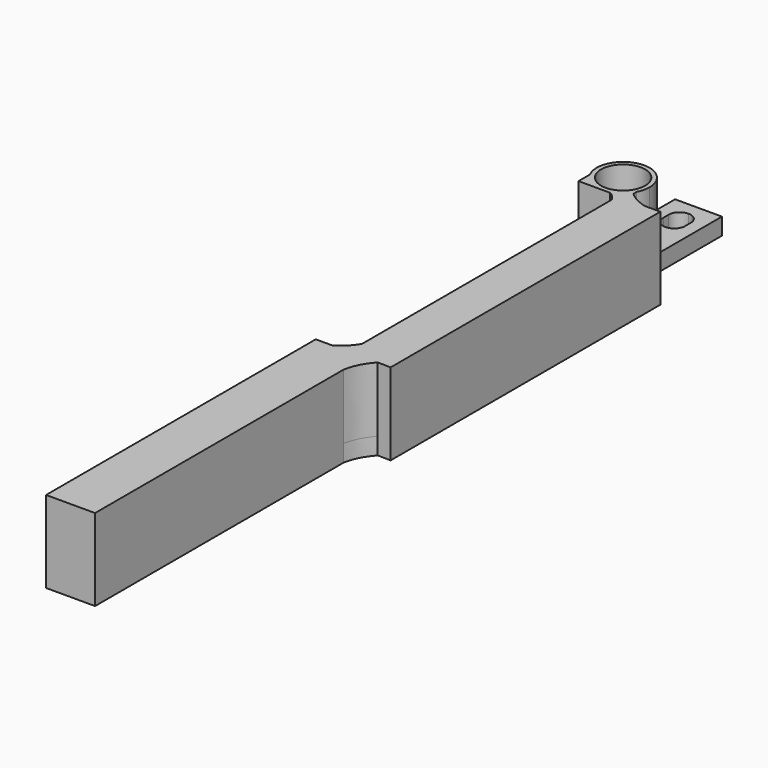
from build123d import *

# Parameters (mm, degrees)
F0_W     = 2.45
F0_H     = 50
F1_DEPTH = 2.5
F2_DEPTH = 9.65
F3_DEPTH = 2.5
F4_DEPTH = 9.65
F5_DEPTH = 9.65
F6_DEPTH = 2.5


with BuildPart() as f1:
    # F0 (on Top) → F1 (new body)
    with BuildSketch(Plane.XY):
        with BuildLine():
            Line((0, 2.1001712409), (0, 0))
            Line((0, 0), (1.025, 0))
            Line((1.025, 0), (1.025, 0.8585484677))
            ThreePointArc((1.025, 0.8585484677), (0.4481513041, 1.426237912), (0, 2.1001712409))
        make_face()
        with BuildLine():
            Line((1.025, 0.8585484677), (1.025, 0))
            Line((1.025, 0), (3.475, 0))
            ThreePointArc((3.475, 0), (2.1769624937, 0.2208504846), (1.025, 0.8585484677))
        make_face()
        with BuildLine():
            ThreePointArc((0, 5.7498287591), (-0.45, 3.925), (0, 2.1001712409))
            Line((0, 2.1001712409), (0, 5.7498287591))
        make_face()
        with BuildLine():
            Line((0, 5.7498287591), (0, 2.1001712409))
            ThreePointArc((0, 2.1001712409), (0.4481513041, 1.426237912), (1.025, 0.8585484677))
            ThreePointArc((1.025, 0.8585484677), (2.1769624937, 0.2208504846), (3.475, 0))
            Line((3.475, 0), (3.475, 0.65))
            ThreePointArc((3.475, 0.65), (0.2, 3.925), (3.475, 7.2))
            Line((3.475, 7.2), (3.475, 7.85))
            ThreePointArc((3.475, 7.85), (1.4448310267, 7.2841723593), (0, 5.7498287591))
        make_face()
        with BuildLine():
            ThreePointArc((5.925, 0.8585484677), (4.7730375063, 0.2208504846), (3.475, 0))
            Line((3.475, 0), (4.7, 0))
            Line((4.7, 0), (5.925, 0))
            Line((5.925, 0), (5.925, 0.8585484677))
        make_face()
        with BuildLine():
            Line((3.475, 0.65), (3.475, 0))
            ThreePointArc((3.475, 0), (4.7730375063, 0.2208504846), (5.925, 0.8585484677))
            ThreePointArc((5.925, 0.8585484677), (6.5018486959, 1.426237912), (6.95, 2.1001712409))
            Line((6.95, 2.1001712409), (6.95, 5.7498287591))
            ThreePointArc((6.95, 5.7498287591), (5.5051689733, 7.2841723593), (3.475, 7.85))
            Line((3.475, 7.85), (3.475, 7.2))
            ThreePointArc((3.475, 7.2), (5.7907747084, 6.2407747084), (6.75, 3.925))
            ThreePointArc((6.75, 3.925), (5.7907747084, 1.6092252916), (3.475, 0.65))
        make_face()
        with BuildLine():
            Line((0, 7.85), (0, 5.7498287591))
            ThreePointArc((0, 5.7498287591), (1.4448310267, 7.2841723593), (3.475, 7.85))
            ThreePointArc((3.475, 7.85), (5.5051689733, 7.2841723593), (6.95, 5.7498287591))
            Line((6.95, 5.7498287591), (6.95, 17.9))
            Line((6.95, 17.9), (3.475, 17.9))
            Line((3.475, 17.9), (0, 17.9))
            Line((0, 17.9), (0, 7.85))
        make_face()
        with BuildLine():
            ThreePointArc((1.8276640256, 14.3833613398), (2.3042302705, 15.55900427), (3.475, 16.0474200003))
            ThreePointArc((3.475, 16.0474200003), (4.5253988967, 15.6691157612), (5.0933824344, 14.7079463483))
            Line((5.0933824344, 14.7079463483), (5.1024433757, 14.1442252627))
            Line((5.1024433757, 14.1442252627), (5.113982201, 13.4263440945))
            ThreePointArc((5.113982201, 13.4263440945), (5.1141409801, 13.4131724726), (5.1141939076, 13.4))
            ThreePointArc((5.1141939076, 13.4), (4.6340851277, 12.2409148723), (3.475, 11.7608060924))
            ThreePointArc((3.475, 11.7608060924), (2.2942628451, 12.2629791393), (1.8369719791, 13.4618131819))
            Line((1.8369719791, 13.4618131819), (1.8276640256, 14.3833613398))
        make_face(mode=Mode.SUBTRACT)
        with BuildLine():
            Line((5.925, 0), (4.7, 0))
            add(Edge.make_bspline(
                [(4.7, 0), (5.2537494339, -0.3164176305), (5.6369397789, -0.7196032093), (5.925, -1.225)],
                knots=[0, 0, 0, 0, 1.7324116139, 1.7324116139, 1.7324116139, 1.7324116139], degree=3))
            Line((5.925, -1.225), (5.925, -0.079424061))
            Line((5.925, -0.079424061), (5.925, 0))
        make_face()
        with BuildLine():
            ThreePointArc((6.95, 2.1001712409), (6.5018486959, 1.426237912), (5.925, 0.8585484677))
            Line((5.925, 0.8585484677), (5.925, 0))
            Line((5.925, 0), (6.95, 0))
            Line((6.95, 0), (6.95, 1.44))
            Line((6.95, 1.44), (6.95, 1.5))
            Line((6.95, 1.5), (6.95, 2.1001712409))
        make_face()
        Polygon((6.95, 0), (5.925, 0), (5.925, -0.079424061), (5.925, -1.225), (5.925, -21.3844068348), (5.925, -22.55), (5.925, -22.9875), (5.925, -25), (9.8284865708, -25), (9.8284865708, -0.079424061), align=None)
        with BuildLine():
            Line((6.95, 5.7498287591), (6.95, 2.1001712409))
            ThreePointArc((6.95, 2.1001712409), (7.2858398025, 2.9852526935), (7.4, 3.925))
            ThreePointArc((7.4, 3.925), (7.2858398025, 4.8647473065), (6.95, 5.7498287591))
        make_face()
        with BuildLine():
            Line((6.95, 1.44), (6.95, 0))
            Line((6.95, 0), (9.8284865708, -0.079424061))
            add(Edge.make_bspline(
                [(6.95, 1.5), (7.7566024847, 0.7003984647), (8.7155010551, 0.2800084476), (9.8284865708, -0.079424061)],
                knots=[0, 0, 0, 0, 3.2833314336, 3.2833314336, 3.2833314336, 3.2833314336], degree=3))
            Line((6.95, 1.5), (6.95, 1.44))
        make_face()
        Polygon((12.1934865708, -0.079424061), (9.8284865708, -0.079424061), (9.8284865708, -25), (9.8284865708, -50.0313035152), (10.2417432854, -50.0397120305), (12.1934865708, -50.079424061), align=None)
        Polygon((9.8284865708, -25), (5.925, -25), (5.925, -26.9515), (5.925, -28.903), (5.925, -47.55), (5.925, -50), (8.29, -50), (9.8284865708, -50.0313035152), align=None)
        with Locations((2.25, -75)):
            Rectangle(F0_W, F0_H)
        with BuildLine():
            Line((10.2417432854, -50.0397120305), (9.8284865708, -50.0313035152))
            Line((9.8284865708, -50.0313035152), (9.8284865708, -50.0397120305))
            Line((9.8284865708, -50.0397120305), (9.8284865708, -50.079424061))
            Line((9.8284865708, -50.079424061), (10.207343012, -50.079424061))
            add(Edge.make_bspline(
                [(10.207343012, -50.079424061), (10.2187605889, -50.0661890592), (10.230227327, -50.0529518896), (10.2417432854, -50.0397120305)],
                knots=[4.2808358806, 4.2808358806, 4.2808358806, 4.2808358806, 4.3292058583, 4.3292058583, 4.3292058583, 4.3292058583], degree=3))
        make_face()
        Polygon((9.8284865708, -50.0397120305), (9.8284865708, -50.0313035152), (8.29, -50), (8.29, -50.0240602729), align=None)
        Polygon((5.925, -50), (3.475, -50), (3.475, -100), (5.925, -100), (5.925, -52.0125), align=None)
        with BuildLine():
            add(Edge.make_bspline(
                [(5.925, -47.55), (5.2342489362, -48.7282052636), (4.4546769932, -49.3181198835), (3.475, -50)],
                knots=[0, 0, 0, 0, 3.4648232278, 3.4648232278, 3.4648232278, 3.4648232278], degree=3))
            Line((3.475, -50), (5.925, -50))
            Line((5.925, -50), (5.925, -47.55))
        make_face()
        with BuildLine():
            Line((9.8284865708, -50.079424061), (9.8284865708, -50.0397120305))
            Line((9.8284865708, -50.0397120305), (8.29, -50.0240602729))
            Line((8.29, -50.0240602729), (8.29, -53.904))
            add(Edge.make_bspline(
                [(8.29, -53.904), (8.5714472143, -52.4050904341), (9.1968655396, -51.250747129), (10.207343012, -50.079424061)],
                knots=[0, 0, 0, 0, 4.2808358806, 4.2808358806, 4.2808358806, 4.2808358806], degree=3))
            Line((10.207343012, -50.079424061), (9.8284865708, -50.079424061))
        make_face()
        Polygon((8.29, -50.0240602729), (8.29, -50), (5.925, -50), align=None)
        Polygon((8.29, -50.0240602729), (5.925, -50), (5.925, -52.0125), (5.925, -100), (8.29, -100), (8.29, -53.904), align=None)
    extrude(amount=-F1_DEPTH)

    # F0 (on Top) → F2 (join)
    with BuildSketch(Plane.XY):
        with BuildLine():
            Line((3.475, 0.65), (3.475, 0))
            ThreePointArc((3.475, 0), (4.7730375063, 0.2208504846), (5.925, 0.8585484677))
            ThreePointArc((5.925, 0.8585484677), (6.5018486959, 1.426237912), (6.95, 2.1001712409))
            Line((6.95, 2.1001712409), (6.95, 5.7498287591))
            ThreePointArc((6.95, 5.7498287591), (5.5051689733, 7.2841723593), (3.475, 7.85))
            Line((3.475, 7.85), (3.475, 7.2))
            ThreePointArc((3.475, 7.2), (5.7907747084, 6.2407747084), (6.75, 3.925))
            ThreePointArc((6.75, 3.925), (5.7907747084, 1.6092252916), (3.475, 0.65))
        make_face()
        with BuildLine():
            Line((0, 5.7498287591), (0, 2.1001712409))
            ThreePointArc((0, 2.1001712409), (0.4481513041, 1.426237912), (1.025, 0.8585484677))
            ThreePointArc((1.025, 0.8585484677), (2.1769624937, 0.2208504846), (3.475, 0))
            Line((3.475, 0), (3.475, 0.65))
            ThreePointArc((3.475, 0.65), (0.2, 3.925), (3.475, 7.2))
            Line((3.475, 7.2), (3.475, 7.85))
            ThreePointArc((3.475, 7.85), (1.4448310267, 7.2841723593), (0, 5.7498287591))
        make_face()
        with BuildLine():
            Line((6.95, 5.7498287591), (6.95, 2.1001712409))
            ThreePointArc((6.95, 2.1001712409), (7.2858398025, 2.9852526935), (7.4, 3.925))
            ThreePointArc((7.4, 3.925), (7.2858398025, 4.8647473065), (6.95, 5.7498287591))
        make_face()
        with BuildLine():
            ThreePointArc((0, 5.7498287591), (-0.45, 3.925), (0, 2.1001712409))
            Line((0, 2.1001712409), (0, 5.7498287591))
        make_face()
        with BuildLine():
            Line((6.95, 1.44), (6.95, 0))
            Line((6.95, 0), (9.8284865708, -0.079424061))
            add(Edge.make_bspline(
                [(6.95, 1.5), (7.7566024847, 0.7003984647), (8.7155010551, 0.2800084476), (9.8284865708, -0.079424061)],
                knots=[0, 0, 0, 0, 3.2833314336, 3.2833314336, 3.2833314336, 3.2833314336], degree=3))
            Line((6.95, 1.5), (6.95, 1.44))
        make_face()
        with BuildLine():
            ThreePointArc((6.95, 2.1001712409), (6.5018486959, 1.426237912), (5.925, 0.8585484677))
            Line((5.925, 0.8585484677), (5.925, 0))
            Line((5.925, 0), (6.95, 0))
            Line((6.95, 0), (6.95, 1.44))
            Line((6.95, 1.44), (6.95, 1.5))
            Line((6.95, 1.5), (6.95, 2.1001712409))
        make_face()
        with BuildLine():
            ThreePointArc((5.925, 0.8585484677), (4.7730375063, 0.2208504846), (3.475, 0))
            Line((3.475, 0), (4.7, 0))
            Line((4.7, 0), (5.925, 0))
            Line((5.925, 0), (5.925, 0.8585484677))
        make_face()
        with BuildLine():
            Line((1.025, 0.8585484677), (1.025, 0))
            Line((1.025, 0), (3.475, 0))
            ThreePointArc((3.475, 0), (2.1769624937, 0.2208504846), (1.025, 0.8585484677))
        make_face()
        with BuildLine():
            Line((0, 2.1001712409), (0, 0))
            Line((0, 0), (1.025, 0))
            Line((1.025, 0), (1.025, 0.8585484677))
            ThreePointArc((1.025, 0.8585484677), (0.4481513041, 1.426237912), (0, 2.1001712409))
        make_face()
        Polygon((6.95, 0), (5.925, 0), (5.925, -0.079424061), (5.925, -1.225), (5.925, -21.3844068348), (5.925, -22.55), (5.925, -22.9875), (5.925, -25), (9.8284865708, -25), (9.8284865708, -0.079424061), align=None)
        with BuildLine():
            Line((5.925, 0), (4.7, 0))
            add(Edge.make_bspline(
                [(4.7, 0), (5.2537494339, -0.3164176305), (5.6369397789, -0.7196032093), (5.925, -1.225)],
                knots=[0, 0, 0, 0, 1.7324116139, 1.7324116139, 1.7324116139, 1.7324116139], degree=3))
            Line((5.925, -1.225), (5.925, -0.079424061))
            Line((5.925, -0.079424061), (5.925, 0))
        make_face()
        Polygon((9.8284865708, -25), (5.925, -25), (5.925, -26.9515), (5.925, -28.903), (5.925, -47.55), (5.925, -50), (8.29, -50), (9.8284865708, -50.0313035152), align=None)
        with BuildLine():
            add(Edge.make_bspline(
                [(5.925, -47.55), (5.2342489362, -48.7282052636), (4.4546769932, -49.3181198835), (3.475, -50)],
                knots=[0, 0, 0, 0, 3.4648232278, 3.4648232278, 3.4648232278, 3.4648232278], degree=3))
            Line((3.475, -50), (5.925, -50))
            Line((5.925, -50), (5.925, -47.55))
        make_face()
        Polygon((8.29, -50.0240602729), (5.925, -50), (5.925, -52.0125), (5.925, -100), (8.29, -100), (8.29, -53.904), align=None)
        Polygon((5.925, -50), (3.475, -50), (3.475, -100), (5.925, -100), (5.925, -52.0125), align=None)
        with Locations((2.25, -75)):
            Rectangle(F0_W, F0_H)
    extrude(amount=F2_DEPTH)

    # F0 (on Top) → F3 (join)
    with BuildSketch(Plane.XY):
        Polygon((12.1934865708, -0.079424061), (9.8284865708, -0.079424061), (9.8284865708, -25), (9.8284865708, -50.0313035152), (10.2417432854, -50.0397120305), (12.1934865708, -50.079424061), align=None)
        Polygon((8.29, -50.0240602729), (5.925, -50), (5.925, -52.0125), (5.925, -100), (8.29, -100), (8.29, -53.904), align=None)
        with BuildLine():
            Line((9.8284865708, -50.079424061), (9.8284865708, -50.0397120305))
            Line((9.8284865708, -50.0397120305), (8.29, -50.0240602729))
            Line((8.29, -50.0240602729), (8.29, -53.904))
            add(Edge.make_bspline(
                [(8.29, -53.904), (8.5714472143, -52.4050904341), (9.1968655396, -51.250747129), (10.207343012, -50.079424061)],
                knots=[0, 0, 0, 0, 4.2808358806, 4.2808358806, 4.2808358806, 4.2808358806], degree=3))
            Line((10.207343012, -50.079424061), (9.8284865708, -50.079424061))
        make_face()
    extrude(amount=-F3_DEPTH)

    # F0 (on Top) → F4 (join)
    with BuildSketch(Plane.XY):
        with BuildLine():
            Line((0, 2.1001712409), (0, 0))
            Line((0, 0), (1.025, 0))
            Line((1.025, 0), (1.025, 0.8585484677))
            ThreePointArc((1.025, 0.8585484677), (0.4481513041, 1.426237912), (0, 2.1001712409))
        make_face()
        with BuildLine():
            Line((1.025, 0.8585484677), (1.025, 0))
            Line((1.025, 0), (3.475, 0))
            ThreePointArc((3.475, 0), (2.1769624937, 0.2208504846), (1.025, 0.8585484677))
        make_face()
        with BuildLine():
            ThreePointArc((0, 5.7498287591), (-0.45, 3.925), (0, 2.1001712409))
            Line((0, 2.1001712409), (0, 5.7498287591))
        make_face()
        with BuildLine():
            Line((0, 5.7498287591), (0, 2.1001712409))
            ThreePointArc((0, 2.1001712409), (0.4481513041, 1.426237912), (1.025, 0.8585484677))
            ThreePointArc((1.025, 0.8585484677), (2.1769624937, 0.2208504846), (3.475, 0))
            Line((3.475, 0), (3.475, 0.65))
            ThreePointArc((3.475, 0.65), (0.2, 3.925), (3.475, 7.2))
            Line((3.475, 7.2), (3.475, 7.85))
            ThreePointArc((3.475, 7.85), (1.4448310267, 7.2841723593), (0, 5.7498287591))
        make_face()
        with BuildLine():
            ThreePointArc((5.925, 0.8585484677), (4.7730375063, 0.2208504846), (3.475, 0))
            Line((3.475, 0), (4.7, 0))
            Line((4.7, 0), (5.925, 0))
            Line((5.925, 0), (5.925, 0.8585484677))
        make_face()
        with BuildLine():
            Line((3.475, 0.65), (3.475, 0))
            ThreePointArc((3.475, 0), (4.7730375063, 0.2208504846), (5.925, 0.8585484677))
            ThreePointArc((5.925, 0.8585484677), (6.5018486959, 1.426237912), (6.95, 2.1001712409))
            Line((6.95, 2.1001712409), (6.95, 5.7498287591))
            ThreePointArc((6.95, 5.7498287591), (5.5051689733, 7.2841723593), (3.475, 7.85))
            Line((3.475, 7.85), (3.475, 7.2))
            ThreePointArc((3.475, 7.2), (5.7907747084, 6.2407747084), (6.75, 3.925))
            ThreePointArc((6.75, 3.925), (5.7907747084, 1.6092252916), (3.475, 0.65))
        make_face()
        with BuildLine():
            Line((5.925, 0), (4.7, 0))
            add(Edge.make_bspline(
                [(4.7, 0), (5.2537494339, -0.3164176305), (5.6369397789, -0.7196032093), (5.925, -1.225)],
                knots=[0, 0, 0, 0, 1.7324116139, 1.7324116139, 1.7324116139, 1.7324116139], degree=3))
            Line((5.925, -1.225), (5.925, -0.079424061))
            Line((5.925, -0.079424061), (5.925, 0))
        make_face()
        with BuildLine():
            ThreePointArc((6.95, 2.1001712409), (6.5018486959, 1.426237912), (5.925, 0.8585484677))
            Line((5.925, 0.8585484677), (5.925, 0))
            Line((5.925, 0), (6.95, 0))
            Line((6.95, 0), (6.95, 1.44))
            Line((6.95, 1.44), (6.95, 1.5))
            Line((6.95, 1.5), (6.95, 2.1001712409))
        make_face()
        Polygon((6.95, 0), (5.925, 0), (5.925, -0.079424061), (5.925, -1.225), (5.925, -21.3844068348), (5.925, -22.55), (5.925, -22.9875), (5.925, -25), (9.8284865708, -25), (9.8284865708, -0.079424061), align=None)
        with BuildLine():
            Line((6.95, 5.7498287591), (6.95, 2.1001712409))
            ThreePointArc((6.95, 2.1001712409), (7.2858398025, 2.9852526935), (7.4, 3.925))
            ThreePointArc((7.4, 3.925), (7.2858398025, 4.8647473065), (6.95, 5.7498287591))
        make_face()
        with BuildLine():
            Line((6.95, 1.44), (6.95, 0))
            Line((6.95, 0), (9.8284865708, -0.079424061))
            add(Edge.make_bspline(
                [(6.95, 1.5), (7.7566024847, 0.7003984647), (8.7155010551, 0.2800084476), (9.8284865708, -0.079424061)],
                knots=[0, 0, 0, 0, 3.2833314336, 3.2833314336, 3.2833314336, 3.2833314336], degree=3))
            Line((6.95, 1.5), (6.95, 1.44))
        make_face()
        Polygon((12.1934865708, -0.079424061), (9.8284865708, -0.079424061), (9.8284865708, -25), (9.8284865708, -50.0313035152), (10.2417432854, -50.0397120305), (12.1934865708, -50.079424061), align=None)
        with BuildLine():
            Line((9.8284865708, -50.079424061), (9.8284865708, -50.0397120305))
            Line((9.8284865708, -50.0397120305), (8.29, -50.0240602729))
            Line((8.29, -50.0240602729), (8.29, -53.904))
            add(Edge.make_bspline(
                [(8.29, -53.904), (8.5714472143, -52.4050904341), (9.1968655396, -51.250747129), (10.207343012, -50.079424061)],
                knots=[0, 0, 0, 0, 4.2808358806, 4.2808358806, 4.2808358806, 4.2808358806], degree=3))
            Line((10.207343012, -50.079424061), (9.8284865708, -50.079424061))
        make_face()
        Polygon((8.29, -50.0240602729), (5.925, -50), (5.925, -52.0125), (5.925, -100), (8.29, -100), (8.29, -53.904), align=None)
    extrude(amount=F4_DEPTH)

    # F0 (on Top) → F5 (join)
    with BuildSketch(Plane.XY):
        with BuildLine():
            Line((0, 2.1001712409), (0, 0))
            Line((0, 0), (1.025, 0))
            Line((1.025, 0), (1.025, 0.8585484677))
            ThreePointArc((1.025, 0.8585484677), (0.4481513041, 1.426237912), (0, 2.1001712409))
        make_face()
        with BuildLine():
            Line((1.025, 0.8585484677), (1.025, 0))
            Line((1.025, 0), (3.475, 0))
            ThreePointArc((3.475, 0), (2.1769624937, 0.2208504846), (1.025, 0.8585484677))
        make_face()
        with BuildLine():
            ThreePointArc((0, 5.7498287591), (-0.45, 3.925), (0, 2.1001712409))
            Line((0, 2.1001712409), (0, 5.7498287591))
        make_face()
        with BuildLine():
            Line((0, 5.7498287591), (0, 2.1001712409))
            ThreePointArc((0, 2.1001712409), (0.4481513041, 1.426237912), (1.025, 0.8585484677))
            ThreePointArc((1.025, 0.8585484677), (2.1769624937, 0.2208504846), (3.475, 0))
            Line((3.475, 0), (3.475, 0.65))
            ThreePointArc((3.475, 0.65), (0.2, 3.925), (3.475, 7.2))
            Line((3.475, 7.2), (3.475, 7.85))
            ThreePointArc((3.475, 7.85), (1.4448310267, 7.2841723593), (0, 5.7498287591))
        make_face()
        with BuildLine():
            ThreePointArc((5.925, 0.8585484677), (4.7730375063, 0.2208504846), (3.475, 0))
            Line((3.475, 0), (4.7, 0))
            Line((4.7, 0), (5.925, 0))
            Line((5.925, 0), (5.925, 0.8585484677))
        make_face()
        with BuildLine():
            Line((3.475, 0.65), (3.475, 0))
            ThreePointArc((3.475, 0), (4.7730375063, 0.2208504846), (5.925, 0.8585484677))
            ThreePointArc((5.925, 0.8585484677), (6.5018486959, 1.426237912), (6.95, 2.1001712409))
            Line((6.95, 2.1001712409), (6.95, 5.7498287591))
            ThreePointArc((6.95, 5.7498287591), (5.5051689733, 7.2841723593), (3.475, 7.85))
            Line((3.475, 7.85), (3.475, 7.2))
            ThreePointArc((3.475, 7.2), (5.7907747084, 6.2407747084), (6.75, 3.925))
            ThreePointArc((6.75, 3.925), (5.7907747084, 1.6092252916), (3.475, 0.65))
        make_face()
        with BuildLine():
            Line((5.925, 0), (4.7, 0))
            add(Edge.make_bspline(
                [(4.7, 0), (5.2537494339, -0.3164176305), (5.6369397789, -0.7196032093), (5.925, -1.225)],
                knots=[0, 0, 0, 0, 1.7324116139, 1.7324116139, 1.7324116139, 1.7324116139], degree=3))
            Line((5.925, -1.225), (5.925, -0.079424061))
            Line((5.925, -0.079424061), (5.925, 0))
        make_face()
        with BuildLine():
            ThreePointArc((6.95, 2.1001712409), (6.5018486959, 1.426237912), (5.925, 0.8585484677))
            Line((5.925, 0.8585484677), (5.925, 0))
            Line((5.925, 0), (6.95, 0))
            Line((6.95, 0), (6.95, 1.44))
            Line((6.95, 1.44), (6.95, 1.5))
            Line((6.95, 1.5), (6.95, 2.1001712409))
        make_face()
        Polygon((6.95, 0), (5.925, 0), (5.925, -0.079424061), (5.925, -1.225), (5.925, -21.3844068348), (5.925, -22.55), (5.925, -22.9875), (5.925, -25), (9.8284865708, -25), (9.8284865708, -0.079424061), align=None)
        with BuildLine():
            Line((6.95, 5.7498287591), (6.95, 2.1001712409))
            ThreePointArc((6.95, 2.1001712409), (7.2858398025, 2.9852526935), (7.4, 3.925))
            ThreePointArc((7.4, 3.925), (7.2858398025, 4.8647473065), (6.95, 5.7498287591))
        make_face()
        with BuildLine():
            Line((6.95, 1.44), (6.95, 0))
            Line((6.95, 0), (9.8284865708, -0.079424061))
            add(Edge.make_bspline(
                [(6.95, 1.5), (7.7566024847, 0.7003984647), (8.7155010551, 0.2800084476), (9.8284865708, -0.079424061)],
                knots=[0, 0, 0, 0, 3.2833314336, 3.2833314336, 3.2833314336, 3.2833314336], degree=3))
            Line((6.95, 1.5), (6.95, 1.44))
        make_face()
        Polygon((12.1934865708, -0.079424061), (9.8284865708, -0.079424061), (9.8284865708, -25), (9.8284865708, -50.0313035152), (10.2417432854, -50.0397120305), (12.1934865708, -50.079424061), align=None)
        Polygon((9.8284865708, -25), (5.925, -25), (5.925, -26.9515), (5.925, -28.903), (5.925, -47.55), (5.925, -50), (8.29, -50), (9.8284865708, -50.0313035152), align=None)
        with Locations((2.25, -75)):
            Rectangle(F0_W, F0_H)
        with BuildLine():
            Line((10.2417432854, -50.0397120305), (9.8284865708, -50.0313035152))
            Line((9.8284865708, -50.0313035152), (9.8284865708, -50.0397120305))
            Line((9.8284865708, -50.0397120305), (9.8284865708, -50.079424061))
            Line((9.8284865708, -50.079424061), (10.207343012, -50.079424061))
            add(Edge.make_bspline(
                [(10.207343012, -50.079424061), (10.2187605889, -50.0661890592), (10.230227327, -50.0529518896), (10.2417432854, -50.0397120305)],
                knots=[4.2808358806, 4.2808358806, 4.2808358806, 4.2808358806, 4.3292058583, 4.3292058583, 4.3292058583, 4.3292058583], degree=3))
        make_face()
        Polygon((9.8284865708, -50.0397120305), (9.8284865708, -50.0313035152), (8.29, -50), (8.29, -50.0240602729), align=None)
        Polygon((5.925, -50), (3.475, -50), (3.475, -100), (5.925, -100), (5.925, -52.0125), align=None)
        with BuildLine():
            add(Edge.make_bspline(
                [(5.925, -47.55), (5.2342489362, -48.7282052636), (4.4546769932, -49.3181198835), (3.475, -50)],
                knots=[0, 0, 0, 0, 3.4648232278, 3.4648232278, 3.4648232278, 3.4648232278], degree=3))
            Line((3.475, -50), (5.925, -50))
            Line((5.925, -50), (5.925, -47.55))
        make_face()
        Polygon((8.29, -50.0240602729), (8.29, -50), (5.925, -50), align=None)
    extrude(amount=F5_DEPTH)

    # F0 (on Top) → F6 (join)
    with BuildSketch(Plane.XY):
        with BuildLine():
            Line((0, 2.1001712409), (0, 0))
            Line((0, 0), (1.025, 0))
            Line((1.025, 0), (1.025, 0.8585484677))
            ThreePointArc((1.025, 0.8585484677), (0.4481513041, 1.426237912), (0, 2.1001712409))
        make_face()
        with BuildLine():
            Line((1.025, 0.8585484677), (1.025, 0))
            Line((1.025, 0), (3.475, 0))
            ThreePointArc((3.475, 0), (2.1769624937, 0.2208504846), (1.025, 0.8585484677))
        make_face()
        with BuildLine():
            ThreePointArc((0, 5.7498287591), (-0.45, 3.925), (0, 2.1001712409))
            Line((0, 2.1001712409), (0, 5.7498287591))
        make_face()
        with BuildLine():
            Line((0, 5.7498287591), (0, 2.1001712409))
            ThreePointArc((0, 2.1001712409), (0.4481513041, 1.426237912), (1.025, 0.8585484677))
            ThreePointArc((1.025, 0.8585484677), (2.1769624937, 0.2208504846), (3.475, 0))
            Line((3.475, 0), (3.475, 0.65))
            ThreePointArc((3.475, 0.65), (0.2, 3.925), (3.475, 7.2))
            Line((3.475, 7.2), (3.475, 7.85))
            ThreePointArc((3.475, 7.85), (1.4448310267, 7.2841723593), (0, 5.7498287591))
        make_face()
        with BuildLine():
            ThreePointArc((5.925, 0.8585484677), (4.7730375063, 0.2208504846), (3.475, 0))
            Line((3.475, 0), (4.7, 0))
            Line((4.7, 0), (5.925, 0))
            Line((5.925, 0), (5.925, 0.8585484677))
        make_face()
        with BuildLine():
            Line((3.475, 0.65), (3.475, 0))
            ThreePointArc((3.475, 0), (4.7730375063, 0.2208504846), (5.925, 0.8585484677))
            ThreePointArc((5.925, 0.8585484677), (6.5018486959, 1.426237912), (6.95, 2.1001712409))
            Line((6.95, 2.1001712409), (6.95, 5.7498287591))
            ThreePointArc((6.95, 5.7498287591), (5.5051689733, 7.2841723593), (3.475, 7.85))
            Line((3.475, 7.85), (3.475, 7.2))
            ThreePointArc((3.475, 7.2), (5.7907747084, 6.2407747084), (6.75, 3.925))
            ThreePointArc((6.75, 3.925), (5.7907747084, 1.6092252916), (3.475, 0.65))
        make_face()
        with BuildLine():
            Line((0, 7.85), (0, 5.7498287591))
            ThreePointArc((0, 5.7498287591), (1.4448310267, 7.2841723593), (3.475, 7.85))
            ThreePointArc((3.475, 7.85), (5.5051689733, 7.2841723593), (6.95, 5.7498287591))
            Line((6.95, 5.7498287591), (6.95, 17.9))
            Line((6.95, 17.9), (3.475, 17.9))
            Line((3.475, 17.9), (0, 17.9))
            Line((0, 17.9), (0, 7.85))
        make_face()
        with BuildLine():
            ThreePointArc((1.8276640256, 14.3833613398), (2.3042302705, 15.55900427), (3.475, 16.0474200003))
            ThreePointArc((3.475, 16.0474200003), (4.5253988967, 15.6691157612), (5.0933824344, 14.7079463483))
            Line((5.0933824344, 14.7079463483), (5.1024433757, 14.1442252627))
            Line((5.1024433757, 14.1442252627), (5.113982201, 13.4263440945))
            ThreePointArc((5.113982201, 13.4263440945), (5.1141409801, 13.4131724726), (5.1141939076, 13.4))
            ThreePointArc((5.1141939076, 13.4), (4.6340851277, 12.2409148723), (3.475, 11.7608060924))
            ThreePointArc((3.475, 11.7608060924), (2.2942628451, 12.2629791393), (1.8369719791, 13.4618131819))
            Line((1.8369719791, 13.4618131819), (1.8276640256, 14.3833613398))
        make_face(mode=Mode.SUBTRACT)
        with BuildLine():
            Line((5.925, 0), (4.7, 0))
            add(Edge.make_bspline(
                [(4.7, 0), (5.2537494339, -0.3164176305), (5.6369397789, -0.7196032093), (5.925, -1.225)],
                knots=[0, 0, 0, 0, 1.7324116139, 1.7324116139, 1.7324116139, 1.7324116139], degree=3))
            Line((5.925, -1.225), (5.925, -0.079424061))
            Line((5.925, -0.079424061), (5.925, 0))
        make_face()
        with BuildLine():
            ThreePointArc((6.95, 2.1001712409), (6.5018486959, 1.426237912), (5.925, 0.8585484677))
            Line((5.925, 0.8585484677), (5.925, 0))
            Line((5.925, 0), (6.95, 0))
            Line((6.95, 0), (6.95, 1.44))
            Line((6.95, 1.44), (6.95, 1.5))
            Line((6.95, 1.5), (6.95, 2.1001712409))
        make_face()
        Polygon((6.95, 0), (5.925, 0), (5.925, -0.079424061), (5.925, -1.225), (5.925, -21.3844068348), (5.925, -22.55), (5.925, -22.9875), (5.925, -25), (9.8284865708, -25), (9.8284865708, -0.079424061), align=None)
        with BuildLine():
            Line((6.95, 5.7498287591), (6.95, 2.1001712409))
            ThreePointArc((6.95, 2.1001712409), (7.2858398025, 2.9852526935), (7.4, 3.925))
            ThreePointArc((7.4, 3.925), (7.2858398025, 4.8647473065), (6.95, 5.7498287591))
        make_face()
        with BuildLine():
            Line((6.95, 1.44), (6.95, 0))
            Line((6.95, 0), (9.8284865708, -0.079424061))
            add(Edge.make_bspline(
                [(6.95, 1.5), (7.7566024847, 0.7003984647), (8.7155010551, 0.2800084476), (9.8284865708, -0.079424061)],
                knots=[0, 0, 0, 0, 3.2833314336, 3.2833314336, 3.2833314336, 3.2833314336], degree=3))
            Line((6.95, 1.5), (6.95, 1.44))
        make_face()
        Polygon((12.1934865708, -0.079424061), (9.8284865708, -0.079424061), (9.8284865708, -25), (9.8284865708, -50.0313035152), (10.2417432854, -50.0397120305), (12.1934865708, -50.079424061), align=None)
        Polygon((9.8284865708, -25), (5.925, -25), (5.925, -26.9515), (5.925, -28.903), (5.925, -47.55), (5.925, -50), (8.29, -50), (9.8284865708, -50.0313035152), align=None)
        with Locations((2.25, -75)):
            Rectangle(F0_W, F0_H)
        with BuildLine():
            Line((10.2417432854, -50.0397120305), (9.8284865708, -50.0313035152))
            Line((9.8284865708, -50.0313035152), (9.8284865708, -50.0397120305))
            Line((9.8284865708, -50.0397120305), (9.8284865708, -50.079424061))
            Line((9.8284865708, -50.079424061), (10.207343012, -50.079424061))
            add(Edge.make_bspline(
                [(10.207343012, -50.079424061), (10.2187605889, -50.0661890592), (10.230227327, -50.0529518896), (10.2417432854, -50.0397120305)],
                knots=[4.2808358806, 4.2808358806, 4.2808358806, 4.2808358806, 4.3292058583, 4.3292058583, 4.3292058583, 4.3292058583], degree=3))
        make_face()
        Polygon((9.8284865708, -50.0397120305), (9.8284865708, -50.0313035152), (8.29, -50), (8.29, -50.0240602729), align=None)
        Polygon((5.925, -50), (3.475, -50), (3.475, -100), (5.925, -100), (5.925, -52.0125), align=None)
        with BuildLine():
            add(Edge.make_bspline(
                [(5.925, -47.55), (5.2342489362, -48.7282052636), (4.4546769932, -49.3181198835), (3.475, -50)],
                knots=[0, 0, 0, 0, 3.4648232278, 3.4648232278, 3.4648232278, 3.4648232278], degree=3))
            Line((3.475, -50), (5.925, -50))
            Line((5.925, -50), (5.925, -47.55))
        make_face()
        with BuildLine():
            Line((9.8284865708, -50.079424061), (9.8284865708, -50.0397120305))
            Line((9.8284865708, -50.0397120305), (8.29, -50.0240602729))
            Line((8.29, -50.0240602729), (8.29, -53.904))
            add(Edge.make_bspline(
                [(8.29, -53.904), (8.5714472143, -52.4050904341), (9.1968655396, -51.250747129), (10.207343012, -50.079424061)],
                knots=[0, 0, 0, 0, 4.2808358806, 4.2808358806, 4.2808358806, 4.2808358806], degree=3))
            Line((10.207343012, -50.079424061), (9.8284865708, -50.079424061))
        make_face()
        Polygon((8.29, -50.0240602729), (8.29, -50), (5.925, -50), align=None)
        Polygon((8.29, -50.0240602729), (5.925, -50), (5.925, -52.0125), (5.925, -100), (8.29, -100), (8.29, -53.904), align=None)
    extrude(amount=-F6_DEPTH)


solid = f1.part
